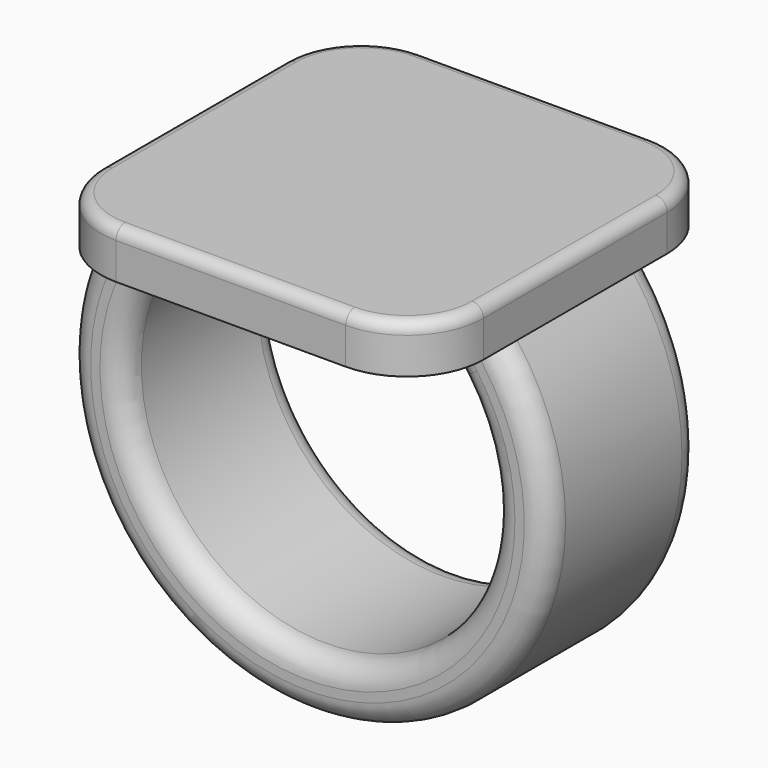
from build123d import *

# Parameters (mm, degrees)
F0_W     = 25.4
F0_H     = 25.4
F1_DEPTH = 3.175
F3_W     = 5.08
F3_H     = 12.7
F6_DEPTH = 6.35
F7_DEPTH = 6.35
F8_R     = 5.08
F9_R     = 1.524
F10_R    = 0.762


with BuildPart() as f1:
    # F0 (on Top) → F1 (new body)
    with BuildSketch(Plane.XY):
        Rectangle(F0_W, F0_H)
    extrude(amount=F1_DEPTH)

    # F4: sweep along a path in F2
    with BuildLine(Plane.XZ) as f4_path:
        ThreePointArc((-10.16, 0), (0, -23.5582897328), (10.16, 0))
    # F3 (on face) → F4 (sweep)
    with BuildSketch(Plane(origin=(0, 0, 0), x_dir=(1, 0, 0), z_dir=(0, 0, -1))):
        with Locations((-10.16, 0)):
            Rectangle(F3_W, F3_H)
    sweep(path=f4_path.line)

    # F5 (on Front) → F6 (join, through all)
    with BuildSketch(Plane.XZ):
        with BuildLine():
            Line((10.0130578512, -2.535746045), (10.16, 0))
            Line((10.16, 0), (7.62, 0))
            ThreePointArc((7.62, 0), (8.9072265211, -1.1822790439), (10.0130578512, -2.535746045))
        make_face()
    extrude(amount=-F6_DEPTH)

    # F7 (add, through all): a face of the model
    f7_faces = [f1.faces().sort_by_distance(p)[0] for p in [
        (9.3051055783, 0, -0.806788918),
    ]]
    extrude(f7_faces, amount=F7_DEPTH)

    # F8
    f8_edges = [f1.edges().sort_by_distance(p)[0] for p in [
        (12.7, -12.7, 1.5875),
        (12.7, 12.7, 1.5875),
        (-12.7, 12.7, 1.5875),
        (-12.7, -12.7, 1.5875),
    ]]
    fillet(f8_edges, radius=F8_R)

    # F9
    f9_edges = [f1.edges().sort_by_distance(p)[0] for p in [
        (-1.743325, -6.35, -21.711017),
        (-1.743325, 6.35, -21.711017),
        (0, 6.35, -25.501344),
        (0, -6.35, -25.501344),
        (8.907227, -6.35, -1.182279),
        (8.907227, 6.35, -1.182279),
    ]]
    fillet(f9_edges, radius=F9_R)

    # F10
    f10_edges = [f1.edges().sort_by_distance(p)[0] for p in [
        (12.7, 0, 3.175),
        (11.212102, -11.212102, 3.175),
        (11.212102, 11.212102, 3.175),
        (0, -12.7, 3.175),
        (0, 12.7, 3.175),
        (-11.212102, -11.212102, 3.175),
        (-11.212102, 11.212102, 3.175),
        (-12.7, 0, 3.175),
    ]]
    fillet(f10_edges, radius=F10_R)


solid = f1.part
